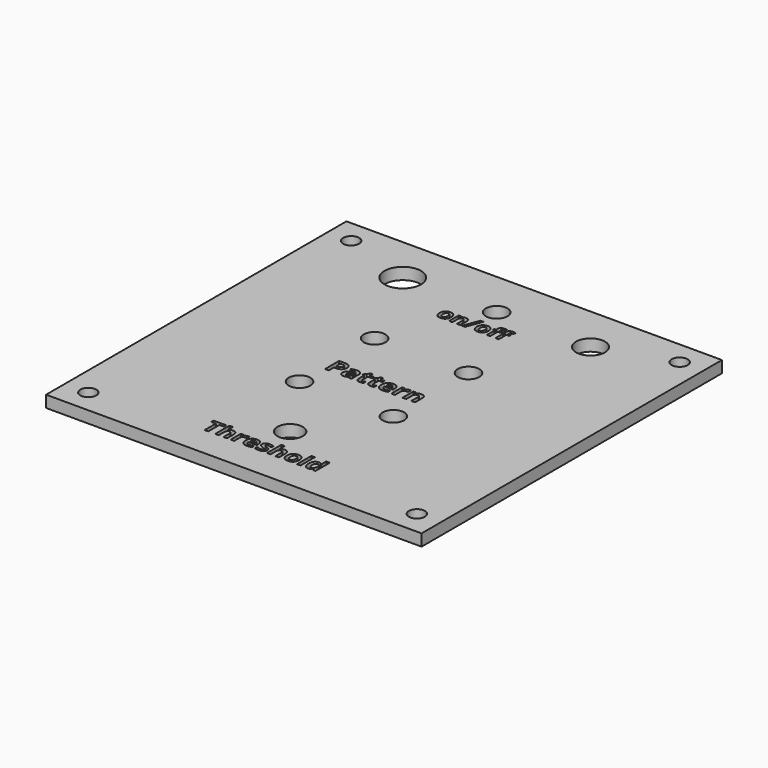
from build123d import *

# Parameters (mm, degrees)
F0_W           = 101.6
F0_H           = 101.6
F0_R           = 2.159
F0_R_2         = 2.921
F0_R_3         = 3.429
F0_R_4         = 4.953
F0_R_5         = 3.937
F1_DEPTH       = 3.175
F2_TEXT_SIZE   = 5.9662344018
F2_TEXT_SIZE_2 = 6.6985330476
F2_TEXT_SIZE_3 = 6.3759021023
F3_DEPTH       = 25.4


# Not quite as in the source:
# - Text() gives the source's letters only with a copy of the font that has no kerning and outlines rounded to 1/6400 em; it was checked with that copy


with BuildPart() as f1:
    # F0 (on Top) → F1 (new body)
    with BuildSketch(Plane.XY):
        with Locations((-34.9792815673, 5.6852983239)):
            Rectangle(F0_W, F0_H)
        with Locations((-79.4292815673, -38.7647016761)):
            Circle(F0_R, mode=Mode.SUBTRACT)
        with Locations((-47.6792815673, -7.0147016761)):
            Circle(F0_R_2, mode=Mode.SUBTRACT)
        with Locations((-34.9792815673, -26.0647016761)):
            Circle(F0_R_3, mode=Mode.SUBTRACT)
        with Locations((9.4707184327, -38.7647016761)):
            Circle(F0_R, mode=Mode.SUBTRACT)
        with Locations((-22.2792815673, -7.0147016761)):
            Circle(F0_R_2, mode=Mode.SUBTRACT)
        with Locations((-47.6792815673, 18.3852983239)):
            Circle(F0_R_2, mode=Mode.SUBTRACT)
        with Locations((-79.4292815673, 50.1352983239)):
            Circle(F0_R, mode=Mode.SUBTRACT)
        with Locations((-60.3792815673, 43.7852983239)):
            Circle(F0_R_4, mode=Mode.SUBTRACT)
        with Locations((-22.2792815673, 18.3852983239)):
            Circle(F0_R_2, mode=Mode.SUBTRACT)
        with Locations((-34.9792815673, 43.7852983239)):
            Circle(F0_R_2, mode=Mode.SUBTRACT)
        with Locations((-9.5792815673, 43.7852983239)):
            Circle(F0_R_5, mode=Mode.SUBTRACT)
        with Locations((9.4707184327, 50.1352983239)):
            Circle(F0_R, mode=Mode.SUBTRACT)
    extrude(amount=F1_DEPTH)

    # F2 (on face) → F3 (cut)
    with BuildSketch(Plane.XY.offset(3.175)):
        with Locations((-44.5042815673, 34.4096095547)):
            Text('on/off', F2_TEXT_SIZE, font='Open Sans', font_style=FontStyle.BOLD, text_align=(TextAlign.LEFT, TextAlign.BOTTOM))
        with Locations((-47.6792815673, 0.8623545296)):
            Text('Pattern', F2_TEXT_SIZE_2, font='Open Sans', font_style=FontStyle.BOLD, text_align=(TextAlign.LEFT, TextAlign.BOTTOM))
        with Locations((-50.8542815673, -36.8223553293)):
            Text('Threshold', F2_TEXT_SIZE_3, font='Open Sans', font_style=FontStyle.BOLD, text_align=(TextAlign.LEFT, TextAlign.BOTTOM))
    extrude(amount=-F3_DEPTH, mode=Mode.SUBTRACT)


solid = f1.part
